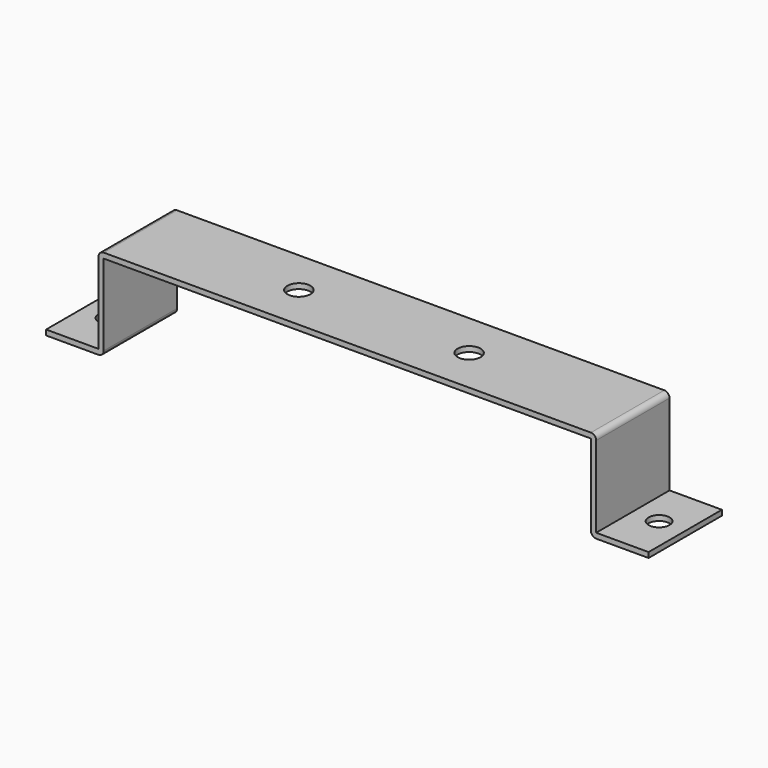
from build123d import *

# Parameters (mm, degrees)
F1_DEPTH = 17.5
F2_R     = 4
F3_DEPTH = 25
F4_R     = 4.4
F5_DEPTH = 25
F6_R     = 2


# Not quite as in the source:
# - a feature names something its author has since deleted; it is built from what else it names


with BuildPart() as f1:
    # F0 (on Front) → F1 (new body, symmetric)
    with BuildSketch(Plane.XZ):
        Polygon((95, -38), (95, -5), (-95, -5), (-95, -38), (-115, -38), (-115, -40), (-93, -40), (-93, -7), (93, -7), (93, -40), (115, -40), (115, -38), align=None)
    extrude(amount=F1_DEPTH, both=True)

    # F2 (on face) → F3 (cut)
    with BuildSketch(Plane.XY.offset(-38)):
        with Locations((-105, 0)):
            Circle(F2_R)
        with Locations((105, 0)):
            Circle(F2_R)
    extrude(amount=-F3_DEPTH, mode=Mode.SUBTRACT)

    # F4 (on face) → F5 (cut)
    with BuildSketch(Plane.XY.offset(-5)):
        with Locations((-32.5, 0)):
            Circle(F4_R)
        with Locations((32.5, 0)):
            Circle(F4_R)
    extrude(amount=-F5_DEPTH, mode=Mode.SUBTRACT)

    # F6
    f6_edges = [f1.edges().sort_by_distance(p)[0] for p in [
        (95, 0, -5),
        (-95, 0, -5),
        (-93, 0, -40),
        (93, 0, -40),
    ]]
    fillet(f6_edges, radius=F6_R)


solid = f1.part
